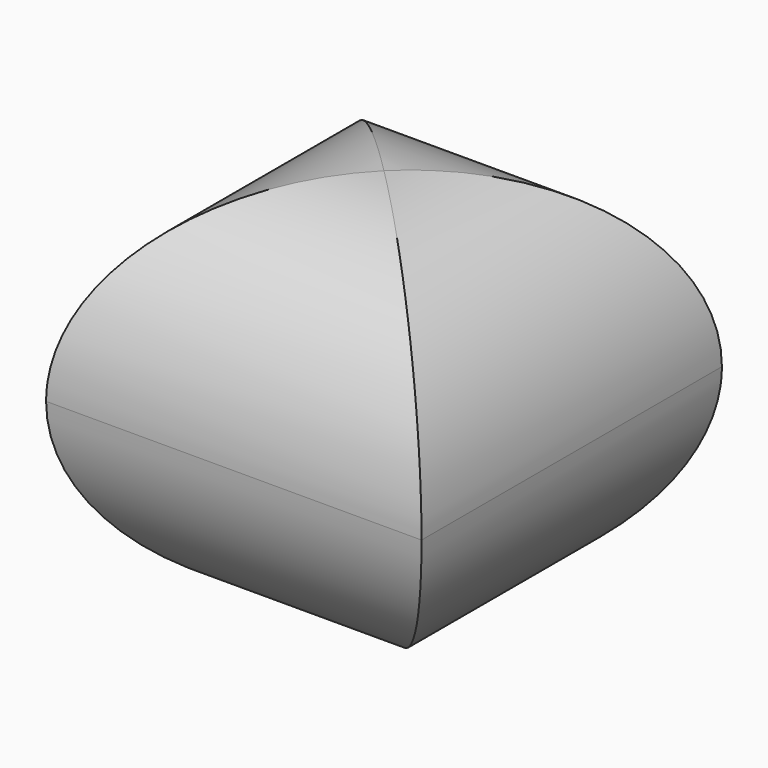
from build123d import *
from build123d import SkipClean  # not in build123d's __all__

# Parameters (mm, degrees)
F0_W     = 304.8
F0_H     = 304.8
F1_DEPTH = 152.4
F2_R     = 152.4
F4_DEPTH = 152.4
F3_R     = 152.4
F5_DEPTH = 152.4


with BuildPart() as f1:
    # F0 (on Top) → F1 (new body, symmetric)
    with BuildSketch(Plane.XY):
        Rectangle(F0_W, F0_H)
    extrude(amount=F1_DEPTH, both=True)

    # F2 (on Right) → F4 (intersect, symmetric)
    with BuildSketch(Plane.YZ):
        Circle(F2_R)
    extrude(amount=F4_DEPTH, both=True, mode=Mode.INTERSECT)

    # F3 (on Front) → F5 (intersect, symmetric)
    with BuildSketch(Plane.XZ):
        Circle(F3_R)
    with SkipClean():  # cleaning this boolean's faces spoils the solid; the shape is the same uncleaned
        extrude(amount=F5_DEPTH, both=True, mode=Mode.INTERSECT)


solid = f1.part
